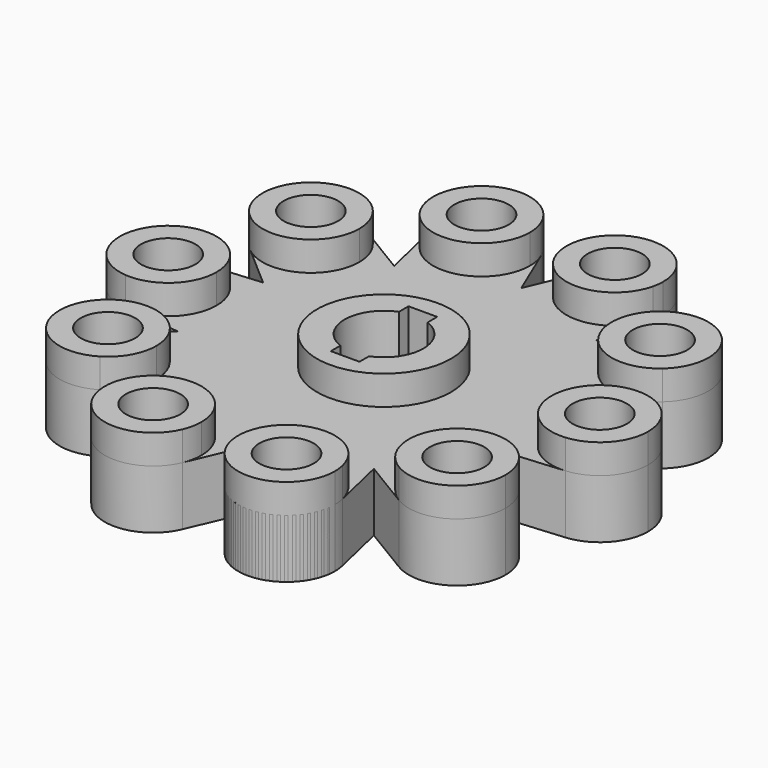
from build123d import *

# Parameters (mm, degrees)
F0_R     = 11.7908412462
F1_DEPTH = 38.1
F0_R_2   = 29.023712578
F2_DEPTH = 25.4


# Not quite as in the source:
# - ends of sketch curves that miss each other by under 0.0002 mm in the source are joined


with BuildPart() as f1:
    # F0 (on Top) → F1 (new body)
    with BuildSketch(Plane.XY):
        with BuildLine():
            ThreePointArc((-64.7426773936, 72.8226518828), (-92.507189101, 67.2104057225), (-89.2650435852, 39.0705068284))
            ThreePointArc((-89.2650435852, 39.0705068284), (-66.8646456266, 35.8659228211), (-54.6352477424, 54.9050670968))
            ThreePointArc((-54.6352477424, 54.9050670968), (-57.3363579251, 65.1909795347), (-64.7426773936, 72.8226518828))
        make_face()
        with Locations((-75.5703416943, 54.9050670968)):
            Circle(F0_R, mode=Mode.SUBTRACT)
    extrude(amount=F1_DEPTH)


with BuildPart() as f1b:
    # F0 (on Top) → F1, piece 2 (new body)
    with BuildSketch(Plane.XY):
        with BuildLine():
            ThreePointArc((-95.1820049773, -20.8599721616), (-79.2470513034, -15.4170941953), (-72.4749854651, 0))
            ThreePointArc((-72.4749854651, 0), (-79.2470520813, 15.4170949099), (-95.1820070823, 20.8599719828))
            ThreePointArc((-95.1820070823, 20.8599719828), (-114.3451733689, -1.0563e-06), (-95.1820049773, -20.8599721616))
        make_face()
        with Locations((-93.410079417, 0)):
            Circle(F0_R, mode=Mode.SUBTRACT)
    extrude(amount=F1_DEPTH)


with BuildPart() as f1c:
    # F0 (on Top) → F1, piece 3 (new body)
    with BuildSketch(Plane.XY):
        with BuildLine():
            ThreePointArc((-54.6352477424, -54.9050670968), (-66.8646465872, -35.8659223818), (-89.265045183, -39.0705082103))
            ThreePointArc((-89.265045183, -39.0705082103), (-92.5071878593, -67.2104074316), (-64.7426755855, -72.8226507902))
            ThreePointArc((-64.7426755855, -72.8226507902), (-57.3363574061, -65.1909786147), (-54.6352477424, -54.9050670968))
        make_face()
        with Locations((-75.5703416943, -54.9050670968)):
            Circle(F0_R, mode=Mode.SUBTRACT)
    extrude(amount=F1_DEPTH)


with BuildPart() as f1d:
    # F0 (on Top) → F1, piece 4 (new body)
    with BuildSketch(Plane.XY):
        with BuildLine():
            ThreePointArc((-7.9302080339, -88.8382647172), (-26.4691132006, -68.0407543354), (-49.2518700311, -84.0773822248))
            ThreePointArc((-49.2518700311, -84.0773822248), (-35.3346007911, -108.7487225658), (-9.5738446427, -96.9695519678))
            ThreePointArc((-9.5738446427, -96.9695519678), (-8.3452309489, -92.9861368721), (-7.9302080339, -88.8382647172))
        make_face()
        with Locations((-28.8653019858, -88.8382647172)):
            Circle(F0_R, mode=Mode.SUBTRACT)
    extrude(amount=F1_DEPTH)


with BuildPart() as f1e:
    # F0 (on Top) → F1, piece 5 (new body)
    with BuildSketch(Plane.XY):
        with BuildLine():
            ThreePointArc((49.2518695507, -84.0773801676), (22.3960011712, -68.9278075214), (9.5738454632, -96.9695539146))
            ThreePointArc((9.5738454632, -96.9695539146), (33.013175176, -109.3583355448), (49.8003959376, -88.8382647172))
            ThreePointArc((49.8003959376, -88.8382647172), (49.6628122466, -86.4420748827), (49.2518695507, -84.0773801676))
        make_face()
        with Locations((28.8653019858, -88.8382647172)):
            Circle(F0_R, mode=Mode.SUBTRACT)
    extrude(amount=F1_DEPTH)


with BuildPart() as f1f:
    # F0 (on Top) → F1, piece 6 (new body)
    with BuildSketch(Plane.XY):
        with BuildLine():
            ThreePointArc((89.2650435852, -39.0705068284), (58.6334942875, -42.5997284711), (64.7426773936, -72.8226518828))
            ThreePointArc((64.7426773936, -72.8226518828), (85.8562541322, -73.1390508659), (96.5054356461, -54.9050670968))
            ThreePointArc((96.5054356461, -54.9050670968), (94.60948597, -46.1993710291), (89.2650435852, -39.0705068284))
        make_face()
        with Locations((75.5703416943, -54.9050670968)):
            Circle(F0_R, mode=Mode.SUBTRACT)
    extrude(amount=F1_DEPTH)


with BuildPart() as f1g:
    # F0 (on Top) → F1, piece 7 (new body)
    with BuildSketch(Plane.XY):
        with BuildLine():
            ThreePointArc((114.3451733689, 0), (108.8271736123, 14.1630281136), (95.1820049773, 20.8599721616))
            ThreePointArc((95.1820049773, 20.8599721616), (72.4749854651, -1.0563e-06), (95.1820070823, -20.8599719828))
            ThreePointArc((95.1820070823, -20.8599719828), (108.8271743269, -14.1630273357), (114.3451733689, 0))
        make_face()
        with Locations((93.410079417, 0)):
            Circle(F0_R, mode=Mode.SUBTRACT)
    extrude(amount=F1_DEPTH)


with BuildPart() as f1h:
    # F0 (on Top) → F1, piece 8 (new body)
    with BuildSketch(Plane.XY):
        Circle(F0_R_2)
        with BuildLine():
            ThreePointArc((-6.209787447, -15.8643485108), (-17.0364026076, 0), (-6.209787447, 15.8643485108))
            Line((-6.209787447, 15.8643485108), (-6.209787447, 21.0346411914))
            Line((-6.209787447, 21.0346411914), (6.209787447, 21.0346411914))
            Line((6.209787447, 21.0346411914), (6.209787447, 15.8643485108))
            ThreePointArc((6.209787447, 15.8643485108), (17.0364026076, 0), (6.209787447, -15.8643485108))
            Line((6.209787447, -15.8643485108), (6.209787447, -21.0346411914))
            Line((6.209787447, -21.0346411914), (-6.209787447, -21.0346411914))
            Line((-6.209787447, -21.0346411914), (-6.209787447, -15.8643485108))
        make_face(mode=Mode.SUBTRACT)
    extrude(amount=F1_DEPTH)


with BuildPart() as f1i:
    # F0 (on Top) → F1, piece 9 (new body)
    with BuildSketch(Plane.XY):
        with BuildLine():
            ThreePointArc((96.5054356461, 54.9050670968), (85.8562532122, 73.1390513849), (64.7426755855, 72.8226507902))
            ThreePointArc((64.7426755855, 72.8226507902), (58.6334955292, 42.599726762), (89.265045183, 39.0705082103))
            ThreePointArc((89.265045183, 39.0705082103), (94.6094864092, 46.1993719898), (96.5054356461, 54.9050670968))
        make_face()
        with Locations((75.5703416943, 54.9050670968)):
            Circle(F0_R, mode=Mode.SUBTRACT)
    extrude(amount=F1_DEPTH)


with BuildPart() as f1j:
    # F0 (on Top) → F1, piece 10 (new body)
    with BuildSketch(Plane.XY):
        with BuildLine():
            ThreePointArc((49.8003959376, 88.8382647172), (33.0131741407, 109.3583357541), (9.5738446427, 96.9695519678))
            ThreePointArc((9.5738446427, 96.9695519678), (22.3960031804, 68.9278068686), (49.2518700311, 84.0773822248))
            ThreePointArc((49.2518700311, 84.0773822248), (49.6628123675, 86.4420759321), (49.8003959376, 88.8382647172))
        make_face()
        with Locations((28.8653019858, 88.8382647172)):
            Circle(F0_R, mode=Mode.SUBTRACT)
    extrude(amount=F1_DEPTH)


with BuildPart() as f1k:
    # F0 (on Top) → F1, piece 11 (new body)
    with BuildSketch(Plane.XY):
        with BuildLine():
            ThreePointArc((-9.5738454632, 96.9695539146), (-35.3346028003, 108.7487219129), (-49.2518695507, 84.0773801676))
            ThreePointArc((-49.2518695507, 84.0773801676), (-26.4691121513, 68.0407544563), (-7.9302080339, 88.8382647172))
            ThreePointArc((-7.9302080339, 88.8382647172), (-8.3452311581, 92.9861379075), (-9.5738454632, 96.9695539146))
        make_face()
        with Locations((-28.8653019858, 88.8382647172)):
            Circle(F0_R, mode=Mode.SUBTRACT)
    extrude(amount=F1_DEPTH)


with BuildPart() as f2:
    # F0 (on Top) → F2 (new body)
    with BuildSketch(Plane.XY):
        with BuildLine():
            ThreePointArc((-95.1820049773, -20.8599721616), (-79.2470513034, -15.4170941953), (-72.4749854651, 0))
            ThreePointArc((-72.4749854651, 0), (-79.2470520813, 15.4170949099), (-95.1820070823, 20.8599719828))
            ThreePointArc((-95.1820070823, 20.8599719828), (-114.3451733689, -1.0563e-06), (-95.1820049773, -20.8599721616))
        make_face()
        with Locations((-93.410079417, 0)):
            Circle(F0_R, mode=Mode.SUBTRACT)
        with BuildLine():
            ThreePointArc((-95.1820070823, 20.8599719828), (-79.2470520813, 15.4170949099), (-72.4749854651, 0))
            ThreePointArc((-72.4749854651, 0), (-79.2470513034, -15.4170941953), (-95.1820049773, -20.8599721616))
            Line((-95.1820049773, -20.8599721616), (-70.6614176311, -22.9809432931))
            Line((-70.6614176311, -22.9809432931), (-89.265045183, -39.0705082103))
            ThreePointArc((-89.265045183, -39.0705082103), (-66.8646465872, -35.8659223818), (-54.6352477424, -54.9050670968))
            ThreePointArc((-54.6352477424, -54.9050670968), (-57.3363574061, -65.1909786147), (-64.7426755855, -72.8226507902))
            Line((-64.7426755855, -72.8226507902), (-43.6584281587, -60.1257128606))
            Line((-43.6584281587, -60.1257128606), (-49.2518700311, -84.0773822248))
            ThreePointArc((-49.2518700311, -84.0773822248), (-26.4691132006, -68.0407543354), (-7.9302080339, -88.8382647172))
            ThreePointArc((-7.9302080339, -88.8382647172), (-8.3452309489, -92.9861368721), (-9.5738446427, -96.9695519678))
            Line((-9.5738446427, -96.9695519678), (0.0205969749, -74.3045037131))
            Line((0.0205969749, -74.3045037131), (9.5738454632, -96.9695539146))
            ThreePointArc((9.5738454632, -96.9695539146), (22.3960011712, -68.9278075214), (49.2518695507, -84.0773801676))
            Line((49.2518695507, -84.0773801676), (43.6917547642, -60.1014996644))
            Line((43.6917547642, -60.1014996644), (64.7426773936, -72.8226518828))
            ThreePointArc((64.7426773936, -72.8226518828), (58.6334942875, -42.5997284711), (89.2650435852, -39.0705068284))
            Line((89.2650435852, -39.0705068284), (70.6741472617, -22.9417655187))
            Line((70.6741472617, -22.9417655187), (95.1820070823, -20.8599719828))
            ThreePointArc((95.1820070823, -20.8599719828), (72.4749854651, -1.0563e-06), (95.1820049773, 20.8599721616))
            Line((95.1820049773, 20.8599721616), (70.6614176311, 22.9809432931))
            Line((70.6614176311, 22.9809432931), (89.265045183, 39.0705082103))
            ThreePointArc((89.265045183, 39.0705082103), (58.6334955292, 42.599726762), (64.7426755855, 72.8226507902))
            Line((64.7426755855, 72.8226507902), (43.6584281587, 60.1257128606))
            Line((43.6584281587, 60.1257128606), (49.2518700311, 84.0773822248))
            ThreePointArc((49.2518700311, 84.0773822248), (22.3960031804, 68.9278068686), (9.5738446427, 96.9695519678))
            Line((9.5738446427, 96.9695519678), (-0.0205969749, 74.3045037131))
            Line((-0.0205969749, 74.3045037131), (-9.5738454632, 96.9695539146))
            ThreePointArc((-9.5738454632, 96.9695539146), (-8.3452311581, 92.9861379075), (-7.9302080339, 88.8382647172))
            ThreePointArc((-7.9302080339, 88.8382647172), (-26.4691121513, 68.0407544563), (-49.2518695507, 84.0773801676))
            Line((-49.2518695507, 84.0773801676), (-43.6917547642, 60.1014996644))
            Line((-43.6917547642, 60.1014996644), (-64.7426773936, 72.8226518828))
            ThreePointArc((-64.7426773936, 72.8226518828), (-57.3363579251, 65.1909795347), (-54.6352477424, 54.9050670968))
            ThreePointArc((-54.6352477424, 54.9050670968), (-66.8646456266, 35.8659228211), (-89.2650435852, 39.0705068284))
            Line((-89.2650435852, 39.0705068284), (-70.6741472617, 22.9417655187))
            Line((-70.6741472617, 22.9417655187), (-95.1820070823, 20.8599719828))
        make_face()
        Circle(F0_R_2, mode=Mode.SUBTRACT)
        with BuildLine():
            ThreePointArc((-64.7426773936, 72.8226518828), (-92.507189101, 67.2104057225), (-89.2650435852, 39.0705068284))
            ThreePointArc((-89.2650435852, 39.0705068284), (-66.8646456266, 35.8659228211), (-54.6352477424, 54.9050670968))
            ThreePointArc((-54.6352477424, 54.9050670968), (-57.3363579251, 65.1909795347), (-64.7426773936, 72.8226518828))
        make_face()
        with Locations((-75.5703416943, 54.9050670968)):
            Circle(F0_R, mode=Mode.SUBTRACT)
        with BuildLine():
            ThreePointArc((-54.6352477424, -54.9050670968), (-66.8646465872, -35.8659223818), (-89.265045183, -39.0705082103))
            ThreePointArc((-89.265045183, -39.0705082103), (-92.5071878593, -67.2104074316), (-64.7426755855, -72.8226507902))
            ThreePointArc((-64.7426755855, -72.8226507902), (-57.3363574061, -65.1909786147), (-54.6352477424, -54.9050670968))
        make_face()
        with Locations((-75.5703416943, -54.9050670968)):
            Circle(F0_R, mode=Mode.SUBTRACT)
        with BuildLine():
            ThreePointArc((-9.5738454632, 96.9695539146), (-35.3346028003, 108.7487219129), (-49.2518695507, 84.0773801676))
            ThreePointArc((-49.2518695507, 84.0773801676), (-26.4691121513, 68.0407544563), (-7.9302080339, 88.8382647172))
            ThreePointArc((-7.9302080339, 88.8382647172), (-8.3452311581, 92.9861379075), (-9.5738454632, 96.9695539146))
        make_face()
        with Locations((-28.8653019858, 88.8382647172)):
            Circle(F0_R, mode=Mode.SUBTRACT)
        with BuildLine():
            ThreePointArc((-7.9302080339, -88.8382647172), (-26.4691132006, -68.0407543354), (-49.2518700311, -84.0773822248))
            ThreePointArc((-49.2518700311, -84.0773822248), (-35.3346007911, -108.7487225658), (-9.5738446427, -96.9695519678))
            ThreePointArc((-9.5738446427, -96.9695519678), (-8.3452309489, -92.9861368721), (-7.9302080339, -88.8382647172))
        make_face()
        with Locations((-28.8653019858, -88.8382647172)):
            Circle(F0_R, mode=Mode.SUBTRACT)
        with BuildLine():
            ThreePointArc((49.8003959376, 88.8382647172), (33.0131741407, 109.3583357541), (9.5738446427, 96.9695519678))
            ThreePointArc((9.5738446427, 96.9695519678), (22.3960031804, 68.9278068686), (49.2518700311, 84.0773822248))
            ThreePointArc((49.2518700311, 84.0773822248), (49.6628123675, 86.4420759321), (49.8003959376, 88.8382647172))
        make_face()
        with Locations((28.8653019858, 88.8382647172)):
            Circle(F0_R, mode=Mode.SUBTRACT)
        with BuildLine():
            ThreePointArc((49.2518695507, -84.0773801676), (22.3960011712, -68.9278075214), (9.5738454632, -96.9695539146))
            ThreePointArc((9.5738454632, -96.9695539146), (33.013175176, -109.3583355448), (49.8003959376, -88.8382647172))
            ThreePointArc((49.8003959376, -88.8382647172), (49.6628122466, -86.4420748827), (49.2518695507, -84.0773801676))
        make_face()
        with Locations((28.8653019858, -88.8382647172)):
            Circle(F0_R, mode=Mode.SUBTRACT)
        with BuildLine():
            ThreePointArc((96.5054356461, 54.9050670968), (85.8562532122, 73.1390513849), (64.7426755855, 72.8226507902))
            ThreePointArc((64.7426755855, 72.8226507902), (58.6334955292, 42.599726762), (89.265045183, 39.0705082103))
            ThreePointArc((89.265045183, 39.0705082103), (94.6094864092, 46.1993719898), (96.5054356461, 54.9050670968))
        make_face()
        with Locations((75.5703416943, 54.9050670968)):
            Circle(F0_R, mode=Mode.SUBTRACT)
        with BuildLine():
            ThreePointArc((89.2650435852, -39.0705068284), (58.6334942875, -42.5997284711), (64.7426773936, -72.8226518828))
            ThreePointArc((64.7426773936, -72.8226518828), (85.8562541322, -73.1390508659), (96.5054356461, -54.9050670968))
            ThreePointArc((96.5054356461, -54.9050670968), (94.60948597, -46.1993710291), (89.2650435852, -39.0705068284))
        make_face()
        with Locations((75.5703416943, -54.9050670968)):
            Circle(F0_R, mode=Mode.SUBTRACT)
        with BuildLine():
            ThreePointArc((114.3451733689, 0), (108.8271736123, 14.1630281136), (95.1820049773, 20.8599721616))
            ThreePointArc((95.1820049773, 20.8599721616), (72.4749854651, -1.0563e-06), (95.1820070823, -20.8599719828))
            ThreePointArc((95.1820070823, -20.8599719828), (108.8271743269, -14.1630273357), (114.3451733689, 0))
        make_face()
        with Locations((93.410079417, 0)):
            Circle(F0_R, mode=Mode.SUBTRACT)
    extrude(amount=F2_DEPTH)


solid = Compound([f1.part, f1b.part, f1c.part, f1d.part, f1e.part, f1f.part, f1g.part, f1h.part, f1i.part, f1j.part, f1k.part, f2.part])
